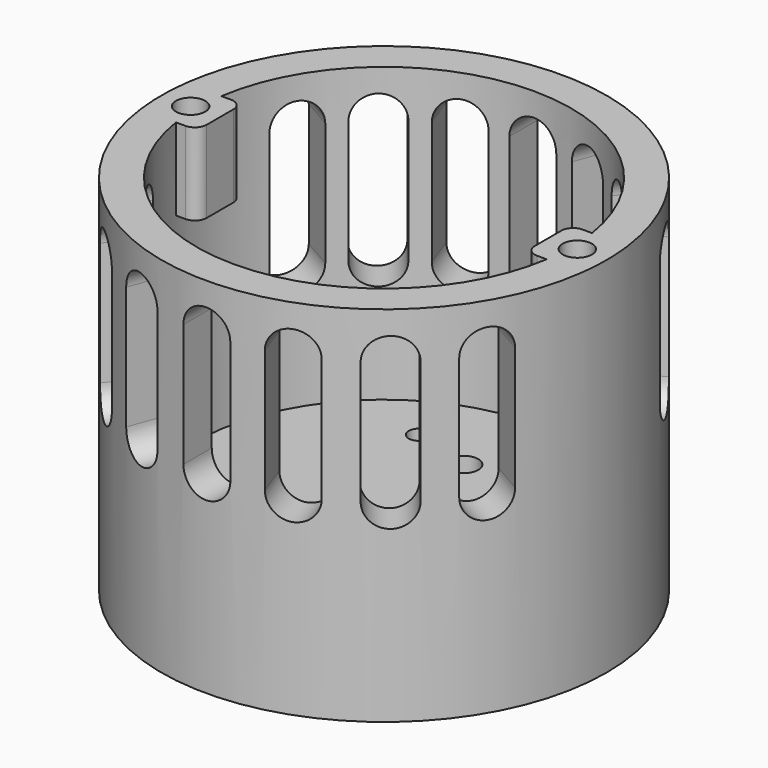
from build123d import *

# Parameters (mm, degrees)
F0_R             = 19
F1_DEPTH         = 6
F2_R             = 19
F2_R_2           = 16
F3_DEPTH         = 25
F5_D             = 2.5
F7_D             = 1.778
F9_DEPTH         = 19.001
F9_COPIES_COUNT  = 4
F9_COPIES_ANGLE  = 60
F9_COPIES1_COUNT = 4
F9_COPIES1_ANGLE = 60
F9_COPIES2_COUNT = 3
F10_W            = 4.8449368961
F10_H            = 4.8449368961
F11_DEPTH        = 7
F13_D            = 2.5
F13_DEPTH        = 6.5
F13_TIP          = 0.7510757738
F14_R            = 1


# Not quite as in the source:
# - a pattern or mirror of a feature is missing from the dataset's text; its kind, count and spacing are read off the source's solid


with BuildPart() as f1:
    # F0 (on Top) → F1 (new body)
    with BuildSketch(Plane.XY):
        Circle(F0_R)
    extrude(amount=F1_DEPTH)

    # F2 (on face) → F3 (join)
    with BuildSketch(Plane.XY.offset(6)):
        Circle(F2_R)
        Circle(F2_R_2, mode=Mode.SUBTRACT)
    extrude(amount=F3_DEPTH)

    # F5 (through all)
    with Locations(Plane(origin=(0, 0, 0), x_dir=(1, 0, 0), z_dir=(0, 0, -1))):
        with Locations((0, -8.5), (0, 8.5)):
            Hole(F5_D / 2)

    # F7 (through all)
    with Locations(Plane.XY.offset(6)):
        with Locations((-5, 10), (4, -10)):
            Hole(F7_D / 2)

    # F8 (on Front) → F9 (cut, through all)
    with BuildSketch(Plane.XZ):
        with BuildLine():
            ThreePointArc((2, 27), (0, 29), (-2, 27))
            Line((-2, 27), (-2, 16.5))
            ThreePointArc((-2, 16.5), (0, 14.5), (2, 16.5))
            Line((2, 16.5), (2, 27))
        make_face()
    f9 = extrude(amount=-F9_DEPTH, mode=Mode.SUBTRACT)

    # F9_copies: F9 ×4 about axis
    f9_copies_axis = Axis((0, 0, 0), (0, 0, 1))
    for i in range(1, F9_COPIES_COUNT):
        add(f9.rotate(f9_copies_axis, i * F9_COPIES_ANGLE / (F9_COPIES_COUNT - 1)), mode=Mode.SUBTRACT)

    # F9_copies1: F9 ×4 about axis
    f9_copies1_axis = Axis((0, 0, 0), (0, 0, -1))
    for i in range(1, F9_COPIES1_COUNT):
        add(f9.rotate(f9_copies1_axis, i * F9_COPIES1_ANGLE / (F9_COPIES1_COUNT - 1)), mode=Mode.SUBTRACT)

    # F9_copies2: F9 ×3 about axis
    f9_copies2_axis = Axis((0, 0, 0), (0, 0, 1))
    for i in range(1, F9_COPIES2_COUNT):
        add(f9.rotate(f9_copies2_axis, i * 360 / F9_COPIES2_COUNT), mode=Mode.SUBTRACT)

    # F9_copies3: F9 across plane
    add(f9.mirror(Plane(origin=(0, 0, 0), x_dir=(-0.984807753, 0.1736481777, 0), z_dir=(-0.1736481777, -0.984807753, 0))), mode=Mode.SUBTRACT)

    # F9_copies4: F9 across plane
    add(f9.mirror(Plane(origin=(0, 0, 0), x_dir=(-0.984807753, -0.1736481777, 0), z_dir=(0.1736481777, -0.984807753, 0))), mode=Mode.SUBTRACT)

    # F9_copies5: F9 across plane
    add(f9.mirror(Plane(origin=(0, 0, 0), x_dir=(-0.9396926208, -0.3420201433, 0), z_dir=(0.3420201433, -0.9396926208, 0))), mode=Mode.SUBTRACT)

    # F9_copies6: F9 across plane
    add(f9.mirror(Plane(origin=(0, 0, 0), x_dir=(0, 0, -1), z_dir=(0, -1, 0))), mode=Mode.SUBTRACT)

    # F9_copies7: F9 across plane
    add(f9.mirror(Plane(origin=(0, 0, 0), x_dir=(-0.9396926208, 0.3420201433, 0), z_dir=(-0.3420201433, -0.9396926208, 0))), mode=Mode.SUBTRACT)

    # F10 (on face) → F11 (join)
    with BuildSketch(Plane.XY.offset(31)):
        with Locations((-16.4224684481, 0)):
            Rectangle(F10_W, F10_H)
    f11 = extrude(amount=-F11_DEPTH)

    # F11_copies: F11 across plane
    add(f11.mirror(Plane(origin=(0, 0, 0), x_dir=(0, 0, 1), z_dir=(1, 0, 0))))

    # F13
    with Locations(Plane.XY.offset(31)):
        with Locations((-16.5, 0), (16.5, 0)):
            Hole(F13_D / 2, depth=F13_DEPTH)
            with Locations((0, 0, -(F13_DEPTH + F13_TIP / 2))):  # 118° drill point
                Cone(0, F13_D / 2, F13_TIP, mode=Mode.SUBTRACT)

    # F14
    f14_edges = [f1.edges().sort_by_distance(p)[0] for p in [
        (-14, 2.422468, 27.5),
        (-14, -2.422468, 27.5),
        (14, 2.422468, 27.5),
        (14, -2.422468, 27.5),
    ]]
    fillet(f14_edges, radius=F14_R)


solid = f1.part
